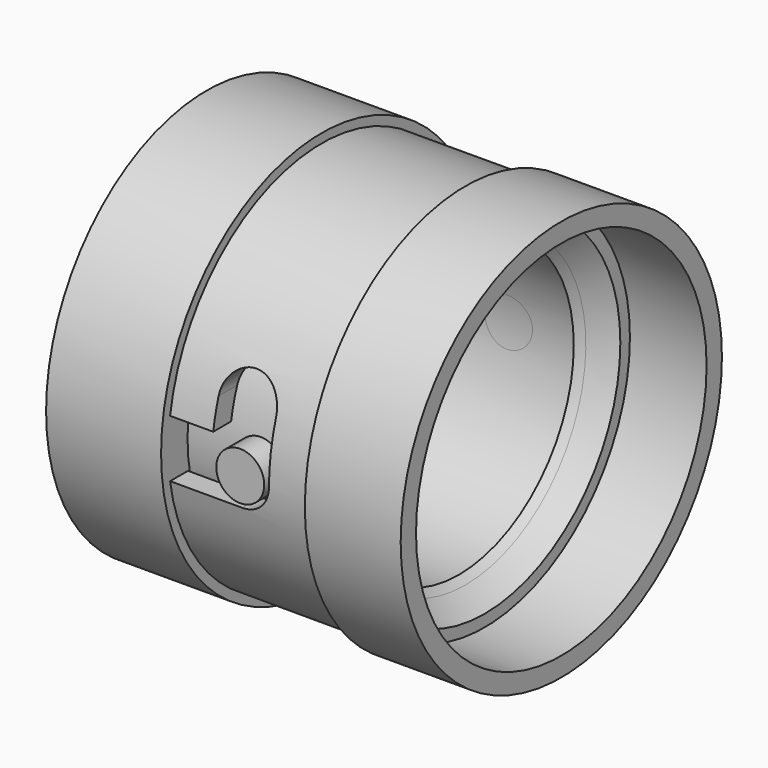
from build123d import *

# Parameters (mm, degrees)
F0_R           = 26.6065
F0_R_2         = 24.0665
F0_R_3         = 19.05
F1_DEPTH       = 2.54
F2_DEPTH       = 12.7
F3_R           = 25.4
F3_R_2         = 22.479
F4_DEPTH       = 19.05
F5_W           = 9.525
F5_H           = 7.62
F6_DEPTH       = 50.8
F6_DEPTH_BACK  = 50.8
F7_R           = 3.81
F8_DEPTH       = 50.8
F8_DEPTH_BACK  = 50.8
F10_DEPTH      = 50.8
F12_DEPTH      = 25.4
F13_R          = 22.225
F13_R_2        = 19.05
F14_DEPTH      = 21.59
F15_START      = -19.05
F13_R_3        = 24.0665
F15_DEPTH      = 2.54
F17_START      = -19.05
F16_R          = 26.6065
F16_R_2        = 24.0665
F17_DEPTH      = 15.24
F18_R          = 3.175
F19_DEPTH      = 25.4
F19_DEPTH_BACK = 25.4
F20_DEPTH      = 25.4
F21_W          = 2.54
F21_H          = 0.889


with BuildPart() as f1:
    # F0 (on Right) → F1 (new body)
    with BuildSketch(Plane.YZ):
        Circle(F0_R)
        Circle(F0_R_2, mode=Mode.SUBTRACT)
        Circle(F0_R_2)
        Circle(F0_R_3, mode=Mode.SUBTRACT)
    extrude(amount=F1_DEPTH)

    # F0 (on Right) → F2 (join)
    with BuildSketch(Plane.YZ):
        Circle(F0_R)
        Circle(F0_R_2, mode=Mode.SUBTRACT)
    extrude(amount=F2_DEPTH)

    # F3 (on Right) → F4 (join)
    with BuildSketch(Plane.YZ):
        Circle(F3_R)
        Circle(F3_R_2, mode=Mode.SUBTRACT)
    extrude(amount=-F4_DEPTH)

    # F5 (on Front) → F6 (cut, two sides)
    with BuildSketch(Plane.XZ) as f6_sk:
        with Locations((-14.2875, 0)):
            Rectangle(F5_W, F5_H)
    extrude(amount=-F6_DEPTH, mode=Mode.SUBTRACT)
    extrude(f6_sk.sketch, amount=F6_DEPTH_BACK, mode=Mode.SUBTRACT)

    # F7 (on Front) → F8 (cut, two sides)
    with BuildSketch(Plane.XZ) as f8_sk:
        with Locations((-9.525, 0)):
            Circle(F7_R)
    extrude(amount=-F8_DEPTH, mode=Mode.SUBTRACT)
    extrude(f8_sk.sketch, amount=F8_DEPTH_BACK, mode=Mode.SUBTRACT)

    # F9 (on Front) → F10 (cut)
    with BuildSketch(Plane.XZ):
        with BuildLine():
            ThreePointArc((-13.335, 7.62), (-9.525, 3.81), (-5.715, 7.62))
            ThreePointArc((-5.715, 7.62), (-9.525, 11.43), (-13.335, 7.62))
        make_face()
        with BuildLine():
            Line((-5.715, 0), (-5.715, 7.62))
            ThreePointArc((-5.715, 7.62), (-9.525, 3.81), (-13.335, 7.62))
            Line((-13.335, 7.62), (-13.335, 0))
            Line((-13.335, 0), (-5.715, 0))
        make_face()
    extrude(amount=F10_DEPTH, mode=Mode.SUBTRACT)

    # F11 (on Front) → F12 (cut)
    with BuildSketch(Plane.XZ):
        with BuildLine():
            ThreePointArc((-13.335, -7.62), (-9.525, -3.81), (-5.715, -7.62))
            Line((-5.715, -7.62), (-5.715, 0))
            Line((-5.715, 0), (-13.335, 0))
            Line((-13.335, 0), (-13.335, -7.62))
        make_face()
        with BuildLine():
            ThreePointArc((-13.335, -7.62), (-9.525, -11.43), (-5.715, -7.62))
            ThreePointArc((-5.715, -7.62), (-9.525, -3.81), (-13.335, -7.62))
        make_face()
    extrude(amount=-F12_DEPTH, mode=Mode.SUBTRACT)


with BuildPart() as f14:
    # F13 (on Right) → F14 (new body)
    with BuildSketch(Plane.YZ):
        Circle(F13_R)
        Circle(F13_R_2, mode=Mode.SUBTRACT)
    extrude(amount=-F14_DEPTH)

    # F13 (on Right) → F15 (join)
    with BuildSketch(Plane.YZ.offset(F15_START)):
        Circle(F13_R_3)
        Circle(F13_R, mode=Mode.SUBTRACT)
    extrude(amount=-F15_DEPTH)

    # F16 (on Right) → F17 (join)
    with BuildSketch(Plane.YZ.offset(F17_START)):
        Circle(F16_R)
        Circle(F16_R_2, mode=Mode.SUBTRACT)
    extrude(amount=-F17_DEPTH)

    # F18 (on Front) → F19 (join, two sides)
    with BuildSketch(Plane.XZ) as f19_sk:
        with Locations((-9.525, 0)):
            Circle(F18_R)
    extrude(amount=F19_DEPTH)
    extrude(f19_sk.sketch, amount=-F19_DEPTH_BACK)

    # F13 (on Right) → F20 (cut)
    with BuildSketch(Plane.YZ):
        Circle(F13_R_2)
    extrude(amount=-F20_DEPTH, mode=Mode.SUBTRACT)


with BuildPart() as f22_tool:
    # F21 (on Front) → F22 (revolve)
    with BuildSketch(Plane.XZ):
        Polygon((0, -19.939), (2.54, -22.479), (2.54, -19.939), align=None)
        with Locations((1.27, -19.4945)):
            Rectangle(F21_W, F21_H)
        Polygon((-0.889, -19.05), (0, -19.939), (0, -19.05), align=None)
    revolve(axis=Axis((12.2344479781, 0, 0), (1, 0, 0)))


with BuildPart() as f1_1:
    add(f1.part)

    # F22: cut by f22_tool
    add(f22_tool.part, mode=Mode.SUBTRACT)

    # F21 (on Front) → F25 (revolve, cut)
    with BuildSketch(Plane.XZ):
        Polygon((0, -19.939), (2.54, -22.479), (2.54, -19.939), align=None)
        with Locations((1.27, -19.4945)):
            Rectangle(F21_W, F21_H)
        Polygon((-0.889, -19.05), (0, -19.939), (0, -19.05), align=None)
    revolve(axis=Axis((12.2344479781, 0, 0), (1, 0, 0)), mode=Mode.SUBTRACT)


with BuildPart() as f14_1:
    add(f14.part)

    # F22: cut by f22_tool
    add(f22_tool.part, mode=Mode.SUBTRACT)

    # F23 (on Front) → F24 (revolve, cut)
    with BuildSketch(Plane.XZ):
        Polygon((-18.161, -19.05), (-21.59, -19.05), (-21.59, -22.479), align=None)
    revolve(axis=Axis((-10.795, 0, 0), (-1, 0, 0)), mode=Mode.SUBTRACT)


solid = Compound([f1_1.part, f14_1.part])
